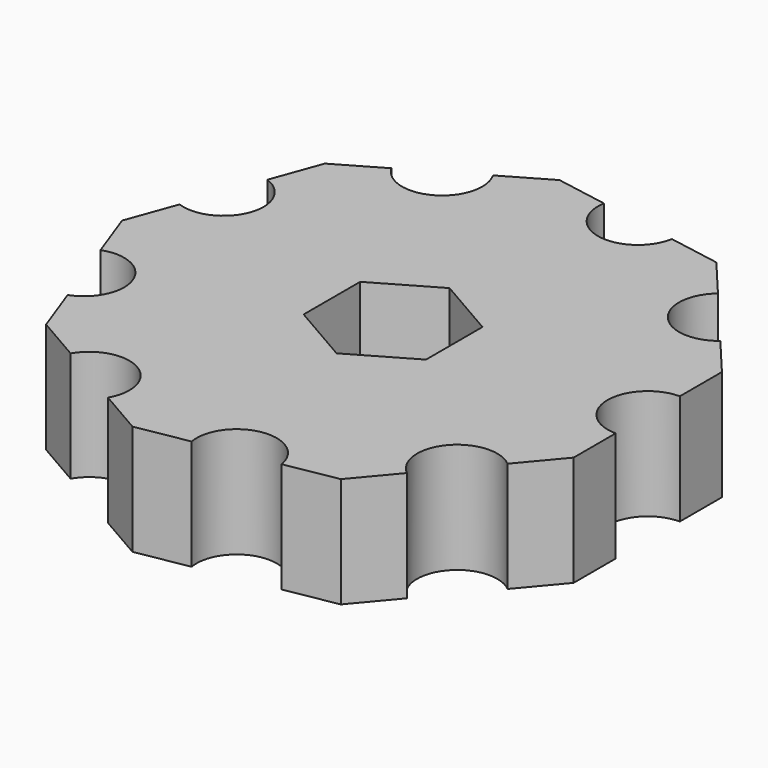
from build123d import *

# Parameters (mm, degrees)
F1_DEPTH        = 5.5
F3_DEPTH        = 4.5
F5_DEPTH        = 25.4
F5_COPIES_COUNT = 9


# Not quite as in the source:
# - a pattern or mirror of a feature is missing from the dataset's text; its kind, count and spacing are read off the source's solid


with BuildPart() as f1:
    # F0 (on Top) → F1 (new body)
    with BuildSketch(Plane.XY):
        Polygon((12.7, -4.6224219752), (12.7, 4.6224219752), (6.7575288552, 11.7043833109), (-2.3468651425, 13.3097336157), (-10.3531348575, 8.6873116405), (-13.5150577104, 0), (-10.3531348575, -8.6873116405), (-2.3468651425, -13.3097336157), (6.7575288552, -11.7043833109), align=None)
    extrude(amount=F1_DEPTH)

    # F2 (on face) → F3 (cut)
    with BuildSketch(Plane.XY.offset(5.5)):
        Polygon((3.05, -1.760918321), (3.05, 1.760918321), (0, 3.5218366421), (-3.05, 1.760918321), (-3.05, -1.760918321), (0, -3.5218366421), align=None)
    extrude(amount=-F3_DEPTH, mode=Mode.SUBTRACT)

    # F4 (on face) → F5 (cut)
    with BuildSketch(Plane.XY.offset(5.5)):
        with BuildLine():
            Line((8.4431892082, -9.6954915293), (11.014339647, -6.6313137568))
            ThreePointArc((11.014339647, -6.6313137568), (8.1966755414, -6.8778274236), (8.4431892082, -9.6954915293))
        make_face()
    f5 = extrude(amount=-F5_DEPTH, mode=Mode.SUBTRACT)

    # F5_copies: F5 ×9 about axis
    f5_copies_axis = Axis((0, 0, 0), (0, 0, 1))
    for i in range(1, F5_COPIES_COUNT):
        add(f5.rotate(f5_copies_axis, i * 360 / F5_COPIES_COUNT), mode=Mode.SUBTRACT)


solid = f1.part
